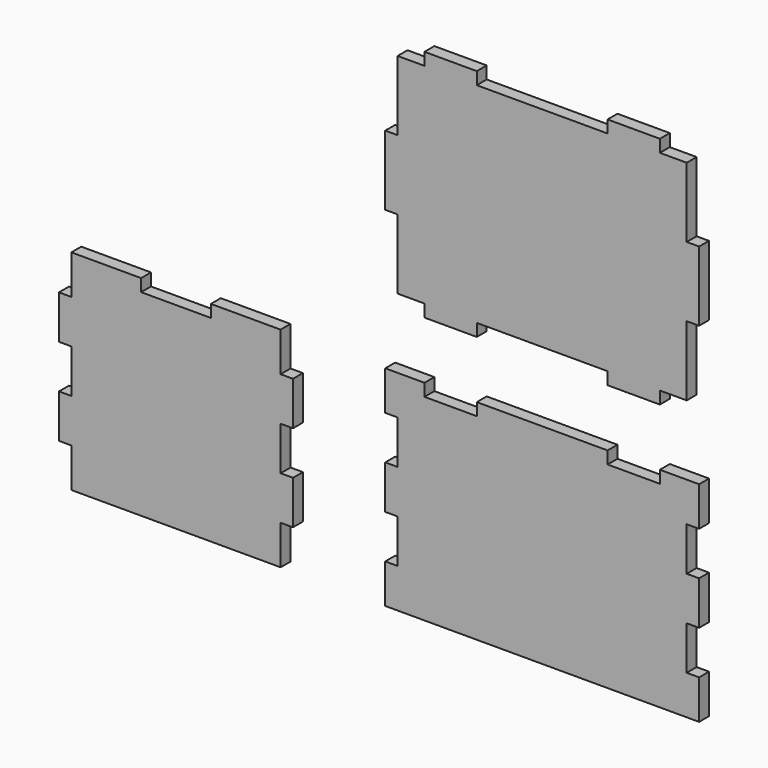
from build123d import *

# Parameters (mm, degrees)
F1_W     = 18.034
F1_H     = 63.5
F2_DEPTH = 18.034
F1_W_2   = 76.2
F1_H_2   = 18.034
F1_H_3   = 101.6


# Not quite as in the source:
# - a variable given as a bare number and used for a length is read in inches; the dataset says mm whatever the document's units were


with BuildPart() as f2:
    # F1 (on Front) → F2 (new body)
    with BuildSketch(Plane.XZ):
        Polygon((-381, 95.25), (-381, 152.4), (-482.6, 152.4), (-482.6, 134.366), (-584.2, 134.366), (-584.2, 152.4), (-685.8, 152.4), (-685.8, 95.25), (-685.8, 31.75), (-685.8, -31.75), (-685.8, -95.25), (-685.8, -152.4), (-381, -152.4), (-381, -95.25), (-381, -31.75), (-381, 31.75), align=None)
        with Locations((-694.817, 63.5)):
            Rectangle(F1_W, F1_H)
        with Locations((-694.817, -63.5)):
            Rectangle(F1_W, F1_H)
        with Locations((-371.983, 63.5)):
            Rectangle(F1_W, F1_H)
        with Locations((-371.983, -63.5)):
            Rectangle(F1_W, F1_H)
    extrude(amount=F2_DEPTH)


with BuildPart() as f2b:
    # F1 (on Front) → F2, piece 2 (new body)
    with BuildSketch(Plane.XZ):
        Polygon((-171.45, 152.4), (-228.6, 152.4), (-228.6, 95.25), (-210.566, 95.25), (-210.566, 31.75), (-228.6, 31.75), (-228.6, -31.75), (-210.566, -31.75), (-210.566, -95.25), (-228.6, -95.25), (-228.6, -152.4), (228.6, -152.4), (228.6, -95.25), (210.566, -95.25), (210.566, -31.75), (228.6, -31.75), (228.6, 31.75), (210.566, 31.75), (210.566, 95.25), (228.6, 95.25), (228.6, 152.4), (171.45, 152.4), (171.45, 134.366), (95.25, 134.366), (95.25, 152.4), (-95.25, 152.4), (-95.25, 134.366), (-171.45, 134.366), align=None)
    extrude(amount=F2_DEPTH)


with BuildPart() as f2c:
    # F1 (on Front) → F2, piece 3 (new body)
    with BuildSketch(Plane.XZ):
        Polygon((-210.566, 254), (-171.45, 254), (-95.25, 254), (95.25, 254), (171.45, 254), (210.566, 254), (210.566, 355.6), (210.566, 457.2), (210.566, 558.8), (171.45, 558.8), (95.25, 558.8), (-95.25, 558.8), (-171.45, 558.8), (-210.566, 558.8), (-210.566, 457.2), (-210.566, 355.6), align=None)
        with Locations((-133.35, 567.817)):
            Rectangle(F1_W_2, F1_H_2)
        with Locations((133.35, 567.817)):
            Rectangle(F1_W_2, F1_H_2)
        with Locations((133.35, 244.983)):
            Rectangle(F1_W_2, F1_H_2)
        with Locations((-133.35, 244.983)):
            Rectangle(F1_W_2, F1_H_2)
        with Locations((-219.583, 406.4)):
            Rectangle(F1_W, F1_H_3)
        with Locations((219.583, 406.4)):
            Rectangle(F1_W, F1_H_3)
    extrude(amount=F2_DEPTH)


solid = Compound([f2.part, f2b.part, f2c.part])
